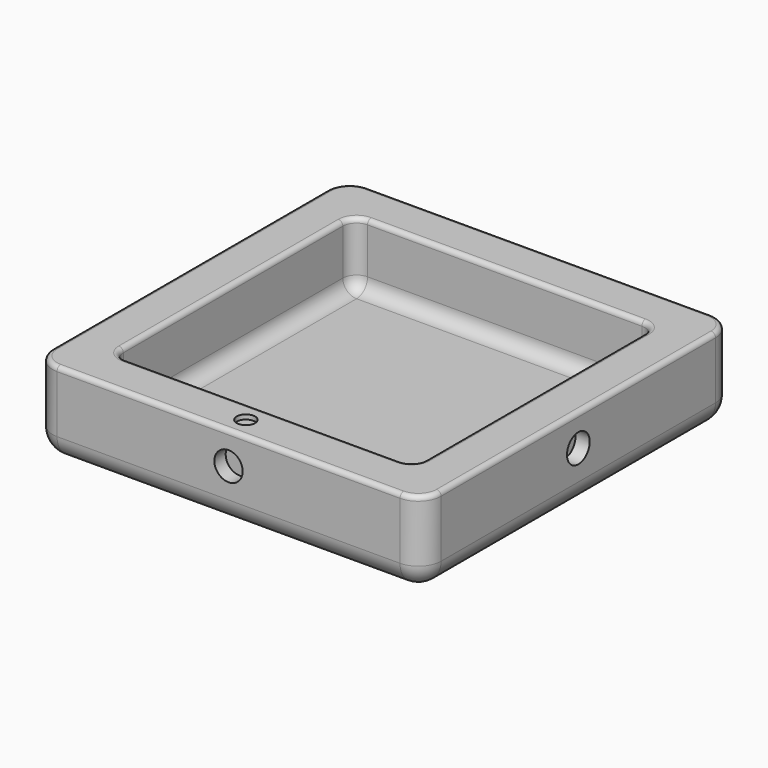
from build123d import *

# Parameters (mm, degrees)
F0_W      = 85
F0_H      = 85
F0_R      = 2
F3_DEPTH  = 18.5
F4_DEPTH  = 14
F5_R      = 5
F6_R      = 3
F7_R      = 1
F8_R      = 3.1
F9_DEPTH  = 3.1
F10_R     = 3.1
F11_DEPTH = 3.1
F12_R     = 3.1
F13_DEPTH = 3.1
F14_R     = 3.1
F15_DEPTH = 3.1
F16_DEPTH = 1
F17_ANGLE = 180


# Not quite as in the source:
# - a feature names something its author has since deleted; it is built from what else it names


with BuildPart() as f3:
    # F0 (on Top) → F3 (new body)
    with BuildSketch(Plane.XY):
        Rectangle(F0_W, F0_H)
        with Locations((0, -37.75)):
            Circle(F0_R, mode=Mode.SUBTRACT)
        with BuildLine():
            ThreePointArc((-33, 30), (-32.1213203436, 32.1213203436), (-30, 33))
            Line((-30, 33), (30, 33))
            ThreePointArc((30, 33), (32.1213203436, 32.1213203436), (33, 30))
            Line((33, 30), (33, -30))
            ThreePointArc((33, -30), (32.1213203436, -32.1213203436), (30, -33))
            Line((30, -33), (-30, -33))
            ThreePointArc((-30, -33), (-32.1213203436, -32.1213203436), (-33, -30))
            Line((-33, -30), (-33, 30))
        make_face(mode=Mode.SUBTRACT)
        with BuildLine():
            Line((30, 33), (-30, 33))
            ThreePointArc((-30, 33), (-32.1213203436, 32.1213203436), (-33, 30))
            Line((-33, 30), (-33, -30))
            ThreePointArc((-33, -30), (-32.1213203436, -32.1213203436), (-30, -33))
            Line((-30, -33), (30, -33))
            ThreePointArc((30, -33), (32.1213203436, -32.1213203436), (33, -30))
            Line((33, -30), (33, 30))
            ThreePointArc((33, 30), (32.1213203436, 32.1213203436), (30, 33))
        make_face()
        with Locations((0, -37.75)):
            Circle(F0_R)
    extrude(amount=F3_DEPTH)

    # F0 (on Top) → F4 (cut)
    with BuildSketch(Plane.XY):
        with BuildLine():
            Line((30, 33), (-30, 33))
            ThreePointArc((-30, 33), (-32.1213203436, 32.1213203436), (-33, 30))
            Line((-33, 30), (-33, -30))
            ThreePointArc((-33, -30), (-32.1213203436, -32.1213203436), (-30, -33))
            Line((-30, -33), (30, -33))
            ThreePointArc((30, -33), (32.1213203436, -32.1213203436), (33, -30))
            Line((33, -30), (33, 30))
            ThreePointArc((33, 30), (32.1213203436, 32.1213203436), (30, 33))
        make_face()
    extrude(amount=F4_DEPTH, mode=Mode.SUBTRACT)

    # F5
    f5_edges = [f3.edges().sort_by_distance(p)[0] for p in [
        (0, 42.5, 18.5),
        (-42.5, 0, 18.5),
        (0, -42.5, 18.5),
        (42.5, 0, 18.5),
        (42.5, 42.5, 9.25),
        (-42.5, 42.5, 9.25),
        (-42.5, -42.5, 9.25),
        (42.5, -42.5, 9.25),
    ]]
    fillet(f5_edges, radius=F5_R)

    # F6
    f6_edges = [f3.edges().sort_by_distance(p)[0] for p in [
        (0, 33, 14),
        (-32.12132, 32.12132, 14),
        (-33, 0, 14),
        (-32.12132, -32.12132, 14),
        (0, -33, 14),
        (32.12132, -32.12132, 14),
        (33, 0, 14),
        (32.12132, 32.12132, 14),
    ]]
    fillet(f6_edges, radius=F6_R)

    # F7
    f7_edges = [f3.edges().sort_by_distance(p)[0] for p in [
        (0, 42.5, 0),
        (41.035534, 41.035534, 0),
        (-41.035534, 41.035534, 0),
        (42.5, 0, 0),
        (-42.5, 0, 0),
        (41.035534, -41.035534, 0),
        (-41.035534, -41.035534, 0),
        (0, -42.5, 0),
        (0, 33, 0),
        (-32.12132, 32.12132, 0),
        (-33, 0, 0),
        (-32.12132, -32.12132, 0),
        (0, -33, 0),
        (32.12132, -32.12132, 0),
        (33, 0, 0),
        (32.12132, 32.12132, 0),
    ]]
    fillet(f7_edges, radius=F7_R)

    # F8 (on face) → F9 (cut)
    with BuildSketch(Plane.XZ.offset(42.5)):
        with Locations((0, 7)):
            Circle(F8_R)
    extrude(amount=-F9_DEPTH, mode=Mode.SUBTRACT)

    # F10 (on face) → F11 (cut)
    with BuildSketch(Plane(origin=(0, 42.5, 0), x_dir=(-1, 0, 0), z_dir=(0, 1, 0))):
        with Locations((0, 7)):
            Circle(F10_R)
    extrude(amount=-F11_DEPTH, mode=Mode.SUBTRACT)

    # F12 (on face) → F13 (cut)
    with BuildSketch(Plane(origin=(-42.5, 0, 0), x_dir=(0, -1, 0), z_dir=(-1, 0, 0))):
        with Locations((0, 7)):
            Circle(F12_R)
    extrude(amount=-F13_DEPTH, mode=Mode.SUBTRACT)

    # F14 (on face) → F15 (cut)
    with BuildSketch(Plane.YZ.offset(42.5)):
        with Locations((0, 7)):
            Circle(F14_R)
    extrude(amount=-F15_DEPTH, mode=Mode.SUBTRACT)

    # F0 (on Top) → F16 (cut)
    with BuildSketch(Plane.XY):
        with Locations((0, -37.75)):
            Circle(F0_R)
    extrude(amount=F16_DEPTH, mode=Mode.SUBTRACT)


with BuildPart() as f3_1:
    # F17: moved
    add(f3.part.rotate(Axis((0, 0, 0), (0, 1, 0)), F17_ANGLE))


solid = f3_1.part
